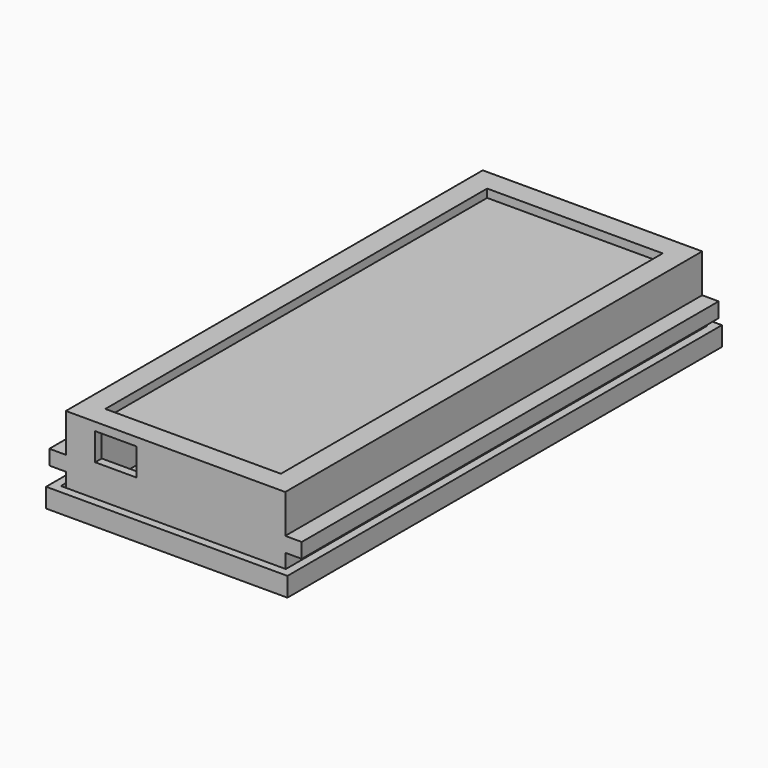
from build123d import *

# Parameters (mm, degrees)
F0_W      = 80
F0_H      = 190
F0_W_2    = 74
F0_H_2    = 184
F1_DEPTH  = 25
F2_W      = 80
F2_H      = 190
F2_W_2    = 64
F2_H_2    = 174
F3_DEPTH  = 3
F6_W      = 88
F6_H      = 198
F6_W_2    = 82
F6_H_2    = 192
F7_DEPTH  = 4
F6_W_3    = 80
F6_H_3    = 190
F6_W_4    = 74
F6_H_4    = 184
F8_DEPTH  = 3
F9_W      = 6.0110352933
F9_H      = 5.4130628705
F10_DEPTH = 190
F11_W     = 15
F11_H     = 10
F12_DEPTH = 3
F13_W     = 64
F13_H     = 174
F14_DEPTH = 1


# Not quite as in the source:
# - a feature names something its author has since deleted; it is built from what else it names


with BuildPart() as f1:
    # F0 (on Top) → F1 (new body)
    with BuildSketch(Plane.XY):
        with Locations((40, 95)):
            Rectangle(F0_W, F0_H)
        with Locations((40, 95)):
            Rectangle(F0_W_2, F0_H_2, mode=Mode.SUBTRACT)
    extrude(amount=F1_DEPTH)

    # F2 (on face) → F3 (join)
    with BuildSketch(Plane.XY.offset(25)):
        with Locations((40, 95)):
            Rectangle(F2_W, F2_H)
        with Locations((40, 95)):
            Rectangle(F2_W_2, F2_H_2, mode=Mode.SUBTRACT)
    extrude(amount=F3_DEPTH)

    # F9 (on face) → F10 (join, through all)
    with BuildSketch(Plane(origin=(0, 190, 0), x_dir=(-1, 0, 0), z_dir=(0, 1, 0))):
        with Locations((3.0055176467, 11.2088900059)):
            Rectangle(F9_W, F9_H)
        with Locations((-83.0055176467, 11.2088900059)):
            Rectangle(F9_W, F9_H)
    extrude(amount=-F10_DEPTH)

    # F11 (on face) → F12 (cut, through all)
    with BuildSketch(Plane.XZ):
        with Locations((18.1946381893, 20)):
            Rectangle(F11_W, F11_H)
    extrude(amount=-F12_DEPTH, mode=Mode.SUBTRACT)


with BuildPart() as f7:
    # F6 (on face) → F7 (new body)
    with BuildSketch(Plane(origin=(0, 0, 0), x_dir=(1, 0, 0), z_dir=(0, 0, -1))):
        with Locations((40, -95)):
            Rectangle(F6_W, F6_H)
        with Locations((40, -95)):
            Rectangle(F6_W_2, F6_H_2, mode=Mode.SUBTRACT)
    extrude(amount=-F7_DEPTH)

    # F6 (on face) → F8 (join)
    with BuildSketch(Plane(origin=(0, 0, 0), x_dir=(1, 0, 0), z_dir=(0, 0, -1))):
        with Locations((40, -95)):
            Rectangle(F6_W, F6_H)
        with Locations((40, -95)):
            Rectangle(F6_W_2, F6_H_2, mode=Mode.SUBTRACT)
        with Locations((40, -95)):
            Rectangle(F6_W_2, F6_H_2)
        with Locations((40, -95)):
            Rectangle(F6_W_3, F6_H_3, mode=Mode.SUBTRACT)
        with Locations((40, -95)):
            Rectangle(F6_W_3, F6_H_3)
        with Locations((40, -95)):
            Rectangle(F6_W_4, F6_H_4, mode=Mode.SUBTRACT)
        with Locations((40, -95)):
            Rectangle(F6_W_4, F6_H_4)
    extrude(amount=F8_DEPTH)


with BuildPart() as f14:
    # F13 (on face) → F14 (new body)
    with BuildSketch(Plane(origin=(0, 0, 25), x_dir=(1, 0, 0), z_dir=(0, 0, -1))):
        with Locations((40, -95)):
            Rectangle(F13_W, F13_H)
    extrude(amount=F14_DEPTH)


solid = Compound([f1.part, f7.part, f14.part])
